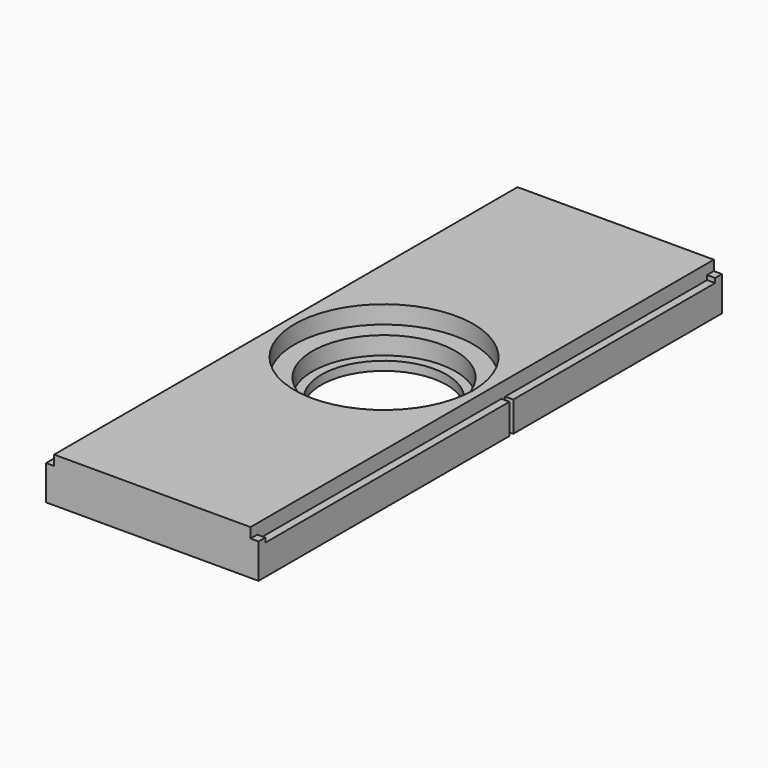
from build123d import *

# Parameters (mm, degrees)
F1_DEPTH      = 64.75
F2_W          = 1.8
F2_H          = 125.7
F3_DEPTH      = 1
F4_R          = 20
F5_DEPTH      = 4
F6_R          = 16
F7_DEPTH      = 4
F8_R          = 14
F9_DEPTH      = 2.001
F10_T         = 2
F10_T3_DEPTH  = 5.9
F10_T5_DEPTH  = 5
F10_T7_DEPTH  = 5.8
F10_T9_DEPTH  = 129.7
F10_T11_DEPTH = 5.9
F10_T13_DEPTH = 5.8
F11_W         = 1.1
F11_H         = 6.75
F12_DEPTH     = 1.9


# Not quite as in the source:
# - a pattern or mirror of a feature is missing from the dataset's text; its kind, count and spacing are read off the source's solid
# - a shell that OpenCascade refuses in one call is made with other operations: the cavity is built on its own and cut out


with BuildPart() as f1:
    # F0 (on Front) → F1 (new body, symmetric)
    with BuildSketch(Plane.XZ):
        Polygon((-23.75, 7.75), (-23.75, 0), (23.75, 0), (23.75, 7.75), (21.95, 7.75), (21.95, 10), (-21.95, 10), (-21.95, 7.75), align=None)
    extrude(amount=F1_DEPTH, both=True)

    # F2 (on face) → F3 (cut)
    with BuildSketch(Plane.XY.offset(7.75)):
        with Locations((22.85, 0)):
            Rectangle(F2_W, F2_H)
    f3 = extrude(amount=-F3_DEPTH, mode=Mode.SUBTRACT)

    # F3_copies: F3 across plane
    add(f3.mirror(Plane(origin=(0, 0, 0), x_dir=(0, 0, -1), z_dir=(-1, 0, 0))), mode=Mode.SUBTRACT)

    # F4 (on face) → F5 (cut)
    with BuildSketch(Plane.XY.offset(10)):
        Circle(F4_R)
    extrude(amount=-F5_DEPTH, mode=Mode.SUBTRACT)

    # F6 (on face) → F7 (cut)
    with BuildSketch(Plane.XY.offset(6)):
        Circle(F6_R)
    extrude(amount=-F7_DEPTH, mode=Mode.SUBTRACT)

    # F8 (on face) → F9 (cut, through all)
    with BuildSketch(Plane.XY.offset(2)):
        Circle(F8_R)
    extrude(amount=-F9_DEPTH, mode=Mode.SUBTRACT)

    # F10: shell of thickness 2, made by hand


with BuildPart() as f10_core1:
    # F10_t2: copy of F1
    add(f1.part)

    # the walls: a layer under each face that stays
    f10_faces = [f10_core1.faces().sort_by_distance(p)[0] for p in [
        (-23.75, 0, 3.875),
        (-22.85, 63.8, 7.75),
        (-22.85, 62.85, 7.25),
        (-22.85, 0, 6.75),
        (-22.85, -62.85, 7.25),
        (-22.85, -63.8, 7.75),
        (0, -64.75, 5),
        (0, 64.75, 5),
        (-21.95, 0, 8.375),
        (23.75, 0, 3.875),
        (22.85, -63.8, 7.75),
        (21.95, 0, 8.375),
        (14.6333333333, 43.1666666667, 10),
        (-14, 0, 1),
        (22.85, 63.8, 7.75),
        (22.85, -62.85, 7.25),
        (22.85, 0, 6.75),
        (22.85, 62.85, 7.25),
        (-20, 0, 8),
        (-10.6666666667, -10.6666666667, 2),
        (-13.3333333333, -13.3333333333, 6),
        (-16, 0, 4),
    ]]
    thicken(f10_faces, amount=-F10_T, mode=Mode.SUBTRACT)

    # F10_s4 → F10_t3 (cut)
    with BuildSketch(Plane.XZ.offset(-66.75)):
        Polygon((-21.97, 7.77), (-21.95, 5.75), (-19.95, 5.75), (-19.95, 7.75), align=None)
        Polygon((21.97, 7.77), (19.95, 7.75), (19.95, 5.75), (21.95, 5.75), align=None)
    extrude(amount=F10_T3_DEPTH, mode=Mode.SUBTRACT)

    # F10_s6 → F10_t5 (cut)
    with BuildSketch(Plane.XY.offset(4.75)):
        Polygon((-21.97, 62.83), (-21.95, 64.85), (-19.95, 64.85), (-19.95, 62.85), align=None)
        Polygon((-21.97, -62.83), (-21.95, -64.85), (-19.95, -64.85), (-19.95, -62.85), align=None)
        Polygon((21.97, -62.83), (19.95, -62.85), (19.95, -64.85), (21.95, -64.85), align=None)
        Polygon((21.97, 62.83), (19.95, 62.85), (19.95, 64.85), (21.95, 64.85), align=None)
    extrude(amount=F10_T5_DEPTH, mode=Mode.SUBTRACT)

    # F10_s8 → F10_t7 (cut)
    with BuildSketch(Plane.YZ.offset(-25.75)):
        Polygon((62.83, 6.77), (64.85, 6.75), (64.85, 4.75), (62.85, 4.75), align=None)
        Polygon((-62.83, 6.77), (-62.85, 4.75), (-64.85, 4.75), (-64.85, 6.75), align=None)
    extrude(amount=F10_T7_DEPTH, mode=Mode.SUBTRACT)

    # F10_s10 → F10_t9 (cut)
    with BuildSketch(Plane.XZ.offset(-64.85)):
        Polygon((-21.97, 6.77), (-21.95, 4.75), (-19.95, 4.75), (-19.95, 6.75), align=None)
        Polygon((21.97, 6.77), (19.95, 6.75), (19.95, 4.75), (21.95, 4.75), align=None)
    extrude(amount=F10_T9_DEPTH, mode=Mode.SUBTRACT)

    # F10_s12 → F10_t11 (cut)
    with BuildSketch(Plane.XZ.offset(60.85)):
        Polygon((-21.97, 7.77), (-21.95, 5.75), (-19.95, 5.75), (-19.95, 7.75), align=None)
        Polygon((21.97, 7.77), (21.95, 5.75), (19.95, 5.75), (19.95, 7.75), align=None)
    extrude(amount=F10_T11_DEPTH, mode=Mode.SUBTRACT)

    # F10_s14 → F10_t13 (cut)
    with BuildSketch(Plane.YZ.offset(19.95)):
        Polygon((-62.83, 6.77), (-64.85, 6.75), (-64.85, 4.75), (-62.85, 4.75), align=None)
        Polygon((62.83, 6.77), (62.85, 4.75), (64.85, 4.75), (64.85, 6.75), align=None)
    extrude(amount=F10_T13_DEPTH, mode=Mode.SUBTRACT)

    # F10_s15 → F10_t16 (revolve, cut)
    with BuildSketch(Plane.XZ):
        Polygon((19.98, 6.02), (22, 6), (22, 4), (20, 4), align=None)
    revolve(axis=Axis((0, 0, 6), (0, 0, 1)), mode=Mode.SUBTRACT)

    # F10_s17 → F10_t18 (revolve, cut)
    with BuildSketch(Plane.XZ):
        Polygon((15.98, 2.02), (16, 0), (18, 0), (18, 2), align=None)
    revolve(axis=Axis((0, 0, 2), (0, 0, 1)), mode=Mode.SUBTRACT)


with BuildPart() as f1_1:
    add(f1.part)

    # what is left inside the walls is the cavity
    f10_cavity = [f10_core1.part.solids().sort_by_distance(p)[0] for p in [
        (0, 20.916667, 0.02),
    ]]
    add(f10_cavity, mode=Mode.SUBTRACT)

    # F11 (on face) → F12 (cut)
    with BuildSketch(Plane.YZ.offset(23.75)):
        with Locations((5.9, 3.375)):
            Rectangle(F11_W, F11_H)
    extrude(amount=-F12_DEPTH, mode=Mode.SUBTRACT)


solid = f1_1.part
